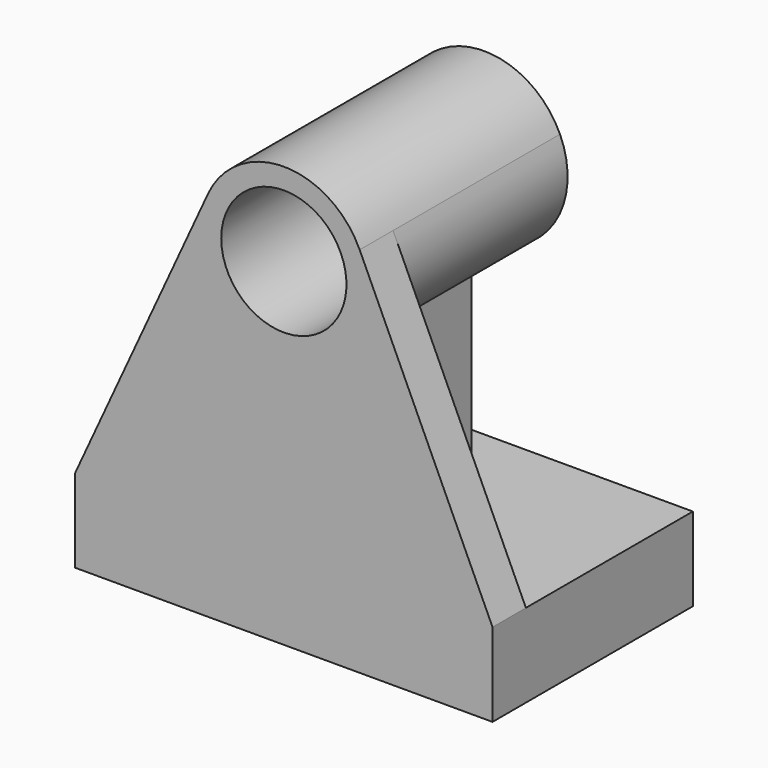
from build123d import *

# Parameters (mm, degrees)
F1_DEPTH = 152.4
F2_R     = 38.1
F3_DEPTH = 152.4
F5_DEPTH = 127
F7_DEPTH = 25.4


with BuildPart() as f1:
    # F0 (on Front) → F1 (new body)
    with BuildSketch(Plane.XZ):
        with BuildLine():
            Line((0, 50.8), (0, 0))
            Line((0, 0), (127, 0))
            Line((127, 0), (127, 154.6394254648))
            ThreePointArc((127, 154.6394254648), (84.2300226684, 178.0283138665), (80.8435975712, 226.6579672344))
            Line((80.8435975712, 226.6579672344), (0, 50.8))
        make_face()
        with BuildLine():
            Line((127, 154.6394254648), (127, 0))
            Line((127, 0), (254, 0))
            Line((254, 0), (254, 50.8))
            Line((254, 50.8), (173.1564024288, 226.6579672344))
            ThreePointArc((173.1564024288, 226.6579672344), (176.6255238934, 216.2997835762), (177.8, 205.4394254648))
            ThreePointArc((177.8, 205.4394254648), (162.9210244843, 169.5184009805), (127, 154.6394254648))
        make_face()
        with BuildLine():
            ThreePointArc((80.8435975712, 226.6579672344), (84.2300226684, 178.0283138665), (127, 154.6394254648))
            ThreePointArc((127, 154.6394254648), (162.9210244843, 169.5184009805), (177.8, 205.4394254648))
            ThreePointArc((177.8, 205.4394254648), (176.6255238934, 216.2997835762), (173.1564024288, 226.6579672344))
            ThreePointArc((173.1564024288, 226.6579672344), (127, 256.2394254648), (80.8435975712, 226.6579672344))
        make_face()
    extrude(amount=F1_DEPTH)

    # F2 (on face) → F3 (cut)
    with BuildSketch(Plane(origin=(0, 0, 0), x_dir=(-1, 0, 0), z_dir=(0, 1, 0))):
        with Locations((-127, 205.4394254648)):
            Circle(F2_R)
    extrude(amount=-F3_DEPTH, mode=Mode.SUBTRACT)

    # F4 (on face) → F5 (cut)
    with BuildSketch(Plane(origin=(0, 0, 0), x_dir=(-1, 0, 0), z_dir=(0, 1, 0))):
        with BuildLine():
            Line((-173.1564024288, 226.6579672344), (-254, 50.8))
            Line((-254, 50.8), (-139.7, 50.8))
            Line((-139.7, 50.8), (-139.7, 156.2525369679))
            ThreePointArc((-139.7, 156.2525369679), (-172.8830053448, 183.6359894848), (-173.1564024288, 226.6579672344))
        make_face()
        with BuildLine():
            Line((0, 50.8), (-80.8435975712, 226.6579672344))
            ThreePointArc((-80.8435975712, 226.6579672344), (-77.3744761066, 216.2997835762), (-76.2, 205.4394254648))
            ThreePointArc((-76.2, 205.4394254648), (-86.8390737159, 174.3309057314), (-114.3, 156.2525369679))
            Line((-114.3, 156.2525369679), (-114.3, 109.0697127324))
            Line((-114.3, 109.0697127324), (-114.3, 50.8))
            Line((-114.3, 50.8), (0, 50.8))
        make_face()
    extrude(amount=-F5_DEPTH, mode=Mode.SUBTRACT)

    # F6 (on face) → F7 (cut)
    with BuildSketch(Plane(origin=(0, 0, 0), x_dir=(-1, 0, 0), z_dir=(0, 1, 0))):
        with BuildLine():
            ThreePointArc((-114.3, 156.2525369679), (-127, 154.6394254648), (-139.7, 156.2525369679))
            Line((-139.7, 156.2525369679), (-139.7, 50.8))
            Line((-139.7, 50.8), (-114.3, 50.8))
            Line((-114.3, 50.8), (-114.3, 156.2525369679))
        make_face()
    extrude(amount=-F7_DEPTH, mode=Mode.SUBTRACT)


solid = f1.part
